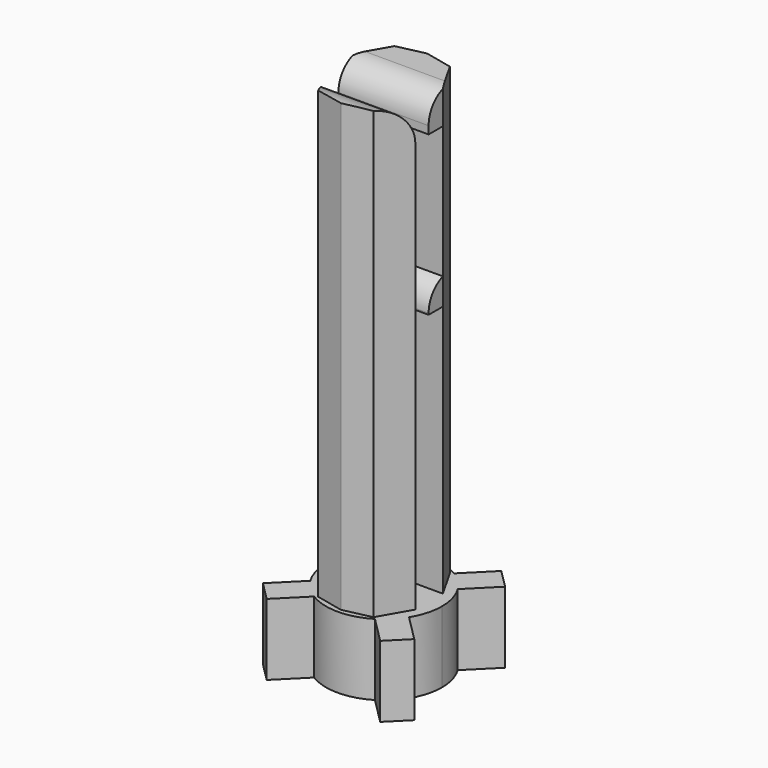
from build123d import *

# Parameters (mm, degrees)
F1_DEPTH     = 4
F3_DEPTH     = 25
F4_R         = 2
F5_W         = 5.058165174
F5_H         = 1.9329627007
F6_DEPTH     = 1
F7_R         = 1.5
F8_W         = 5.058165174
F8_H         = 1.4937128872
F9_DEPTH     = 1
F10_T1_DEPTH = 12.1292329858


# Not quite as in the source:
# - a fillet or chamfer that OpenCascade refuses, or shapes differently, is made with other operations: its cross-section is extruded or revolved along the edge and cut away or added


with BuildPart() as f1:
    # F0 (on Top) → F1 (new body)
    with BuildSketch(Plane.XY):
        with BuildLine():
            ThreePointArc((2.7663980634, -1.7057378916), (3.1267629992, -0.8864835853), (3.25, 0))
            ThreePointArc((3.25, 0), (3.1267629992, 0.8864835853), (2.7663980634, 1.7057378916))
            ThreePointArc((2.7663980634, 1.7057378916), (2.2980970389, 2.2980970389), (1.7057378916, 2.7663980634))
            ThreePointArc((1.7057378916, 2.7663980634), (0, 3.25), (-1.7057378916, 2.7663980634))
            ThreePointArc((-1.7057378916, 2.7663980634), (-2.2980970389, 2.2980970389), (-2.7663980634, 1.7057378916))
            ThreePointArc((-2.7663980634, 1.7057378916), (-3.25, 0), (-2.7663980634, -1.7057378916))
            ThreePointArc((-2.7663980634, -1.7057378916), (-2.2980970389, -2.2980970389), (-1.7057378916, -2.7663980634))
            ThreePointArc((-1.7057378916, -2.7663980634), (0, -3.25), (1.7057378916, -2.7663980634))
            ThreePointArc((1.7057378916, -2.7663980634), (2.2980970389, -2.2980970389), (2.7663980634, -1.7057378916))
        make_face()
        with BuildLine():
            ThreePointArc((1.7057378916, 2.7663980634), (2.2980970389, 2.2980970389), (2.7663980634, 1.7057378916))
            Line((2.7663980634, 1.7057378916), (4.2426406871, 3.1819805153))
            Line((4.2426406871, 3.1819805153), (3.7123106012, 3.7123106012))
            Line((3.7123106012, 3.7123106012), (3.1819805153, 4.2426406871))
            Line((3.1819805153, 4.2426406871), (1.7057378916, 2.7663980634))
        make_face()
        with BuildLine():
            Line((4.2426406871, -3.1819805153), (2.7663980634, -1.7057378916))
            ThreePointArc((2.7663980634, -1.7057378916), (2.2980970389, -2.2980970389), (1.7057378916, -2.7663980634))
            Line((1.7057378916, -2.7663980634), (3.1819805153, -4.2426406871))
            Line((3.1819805153, -4.2426406871), (3.7123106012, -3.7123106012))
            Line((3.7123106012, -3.7123106012), (4.2426406871, -3.1819805153))
        make_face()
        with BuildLine():
            ThreePointArc((-2.7663980634, 1.7057378916), (-2.2980970389, 2.2980970389), (-1.7057378916, 2.7663980634))
            Line((-1.7057378916, 2.7663980634), (-3.1819805153, 4.2426406871))
            Line((-3.1819805153, 4.2426406871), (-3.7123106012, 3.7123106012))
            Line((-3.7123106012, 3.7123106012), (-4.2426406871, 3.1819805153))
            Line((-4.2426406871, 3.1819805153), (-2.7663980634, 1.7057378916))
        make_face()
        with BuildLine():
            Line((-3.1819805153, -4.2426406871), (-1.7057378916, -2.7663980634))
            ThreePointArc((-1.7057378916, -2.7663980634), (-2.2980970389, -2.2980970389), (-2.7663980634, -1.7057378916))
            Line((-2.7663980634, -1.7057378916), (-4.2426406871, -3.1819805153))
            Line((-4.2426406871, -3.1819805153), (-3.7123106012, -3.7123106012))
            Line((-3.7123106012, -3.7123106012), (-3.1819805153, -4.2426406871))
        make_face()
    extrude(amount=F1_DEPTH)

    # F2 (on face) → F3 (join)
    with BuildSketch(Plane.XY.offset(4)):
        Polygon((-1.5528574586, 2.6730068494), (-2.529082587, 0.9646130493), (2.529082587, 0.9646130493), (1.5528574586, 2.6730068494), (0, 3.0187531374), align=None)
        Polygon((2.529082587, -0.9646130493), (-2.529082587, -0.9646130493), (-1.5528574586, -2.6730068494), (0, -3.0187531374), (1.5528574586, -2.6730068494), align=None)
    extrude(amount=F3_DEPTH)

    # F4
    f4_edges = [f1.edges().sort_by_distance(p)[0] for p in [
        (0, -0.964613, 29),
    ]]
    fillet(f4_edges, radius=F4_R)

    # F5 (on face) → F6 (join)
    with BuildSketch(Plane.XZ.offset(-0.9646130493)):
        with Locations((0, 28.0335186496)):
            Rectangle(F5_W, F5_H)
    extrude(amount=F6_DEPTH)

    # F7
    f7_edges = [f1.edges().sort_by_distance(p)[0] for p in [
        (0, -0.035387, 29),
    ]]
    fillet(f7_edges, radius=F7_R)

    # F8 (on face) → F9 (join)
    with BuildSketch(Plane.XZ.offset(-0.9646130493)):
        with Locations((0, 18.9132643864)):
            Rectangle(F8_W, F8_H)
    extrude(amount=F9_DEPTH)

    # F10: fillet of radius 1.5 on 1 edges, made by hand

    # F10_s2 → F10_t1 (cut)
    with BuildSketch(Plane.YZ.offset(-6.0646164929)):
        with BuildLine():
            ThreePointArc((0.9646130493, 19.6601208299), (0.2398681779, 19.1119326714), (-0.0353869507, 18.2459072676))
            Line((-0.0353869507, 18.2459072676), (-0.0353869507, 19.6601208299))
            Line((-0.0353869507, 19.6601208299), (0.9646130493, 19.6601208299))
        make_face()
    extrude(amount=F10_T1_DEPTH, mode=Mode.SUBTRACT)


solid = f1.part
